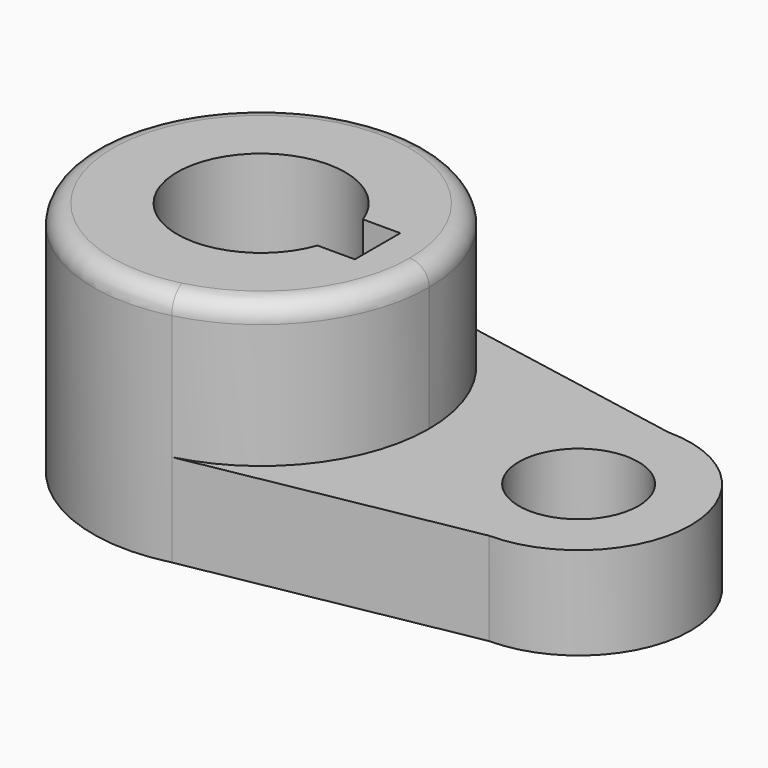
from build123d import *

# Parameters (mm, degrees)
F1_DEPTH = 40.2336
F0_R     = 10.16
F2_DEPTH = 15.7734
F3_R     = 3.302


# Not quite as in the source:
# - a feature names something its author has since deleted; it is built from what else it names


with BuildPart() as f1:
    # F0 (on Top) → F1 (new body)
    with BuildSketch(Plane.XY):
        with BuildLine():
            ThreePointArc((6.9836113022, -27.7084788139), (22.5398238454, -17.5637970274), (28.575, 0))
            ThreePointArc((28.575, 0), (22.1437005793, 18.0606519721), (5.7447533049, 27.9915779203))
            ThreePointArc((5.7447533049, 27.9915779203), (-28.5679347598, -0.6353963805), (6.9836113022, -27.7084788139))
        make_face()
        with BuildLine():
            ThreePointArc((13.4477648793, -4.826), (-14.2875, 0), (13.4477648793, 4.826))
            Line((13.4477648793, 4.826), (19.7977648793, 4.826))
            Line((19.7977648793, 4.826), (19.7977648793, -4.826))
            Line((19.7977648793, -4.826), (13.4477648793, -4.826))
        make_face(mode=Mode.SUBTRACT)
    extrude(amount=F1_DEPTH)

    # F0 (on Top) → F2 (join)
    with BuildSketch(Plane.XY):
        with BuildLine():
            ThreePointArc((5.7447533049, 27.9915779203), (22.1437005793, 18.0606519721), (28.575, 0))
            ThreePointArc((28.575, 0), (22.5398238454, -17.5637970274), (6.9836113022, -27.7084788139))
            Line((6.9836113022, -27.7084788139), (53.975, -19.05))
            ThreePointArc((53.975, -19.05), (34.925, 0), (53.975, 19.05))
            Line((53.975, 19.05), (5.7447533049, 27.9915779203))
        make_face()
        with BuildLine():
            ThreePointArc((73.025, 0), (67.4453841816, 13.4703841816), (53.975, 19.05))
            ThreePointArc((53.975, 19.05), (34.925, 0), (53.975, -19.05))
            ThreePointArc((53.975, -19.05), (67.4453841816, -13.4703841816), (73.025, 0))
        make_face()
        with Locations((53.975, 0)):
            Circle(F0_R, mode=Mode.SUBTRACT)
    extrude(amount=F2_DEPTH)

    # F3
    f3_edges = [f1.edges().sort_by_distance(p)[0] for p in [
        (-6.983611, 27.708479, 40.2336),
    ]]
    fillet(f3_edges, radius=F3_R)


solid = f1.part
